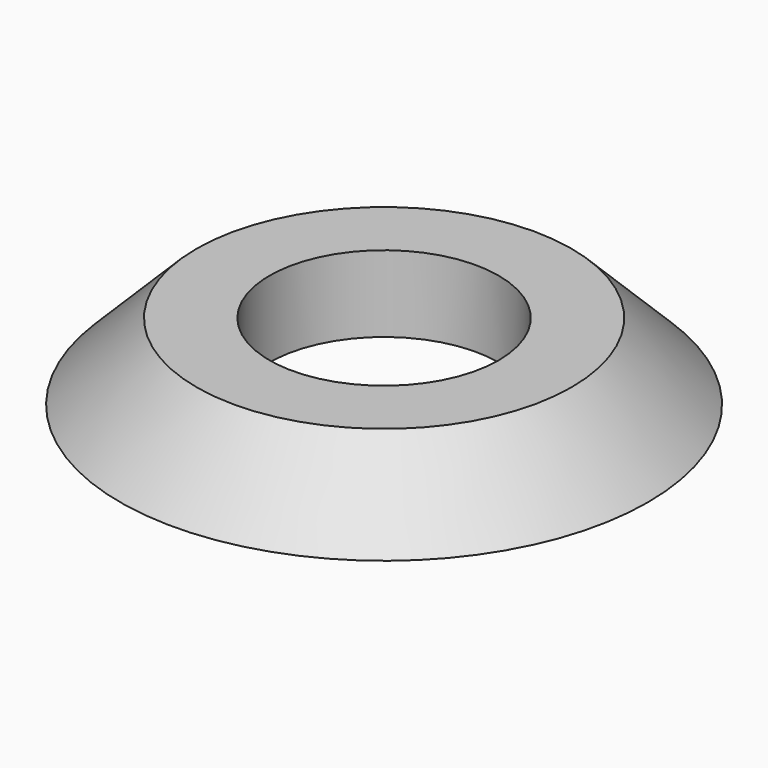
from build123d import *

# Parameters (mm, degrees)
F0_R     = 19
F0_R_2   = 8.25
F1_DEPTH = 5.5
F2_SIZE  = 5.49999


# Not quite as in the source:
# - a fillet or chamfer is up to 0.001 mm smaller than in the source, because OpenCascade refuses the exact size


with BuildPart() as f1:
    # F0 (on Top) → F1 (new body)
    with BuildSketch(Plane.XY):
        Circle(F0_R)
        Circle(F0_R_2, mode=Mode.SUBTRACT)
    extrude(amount=F1_DEPTH)

    # F2 (size 5.5 in the source; OpenCascade refuses exactly that, so slightly less here)
    f2_edges = [f1.edges().sort_by_distance(p)[0] for p in [
        (-19, 0, 5.5),
    ]]
    chamfer(f2_edges, length=F2_SIZE)


solid = f1.part
